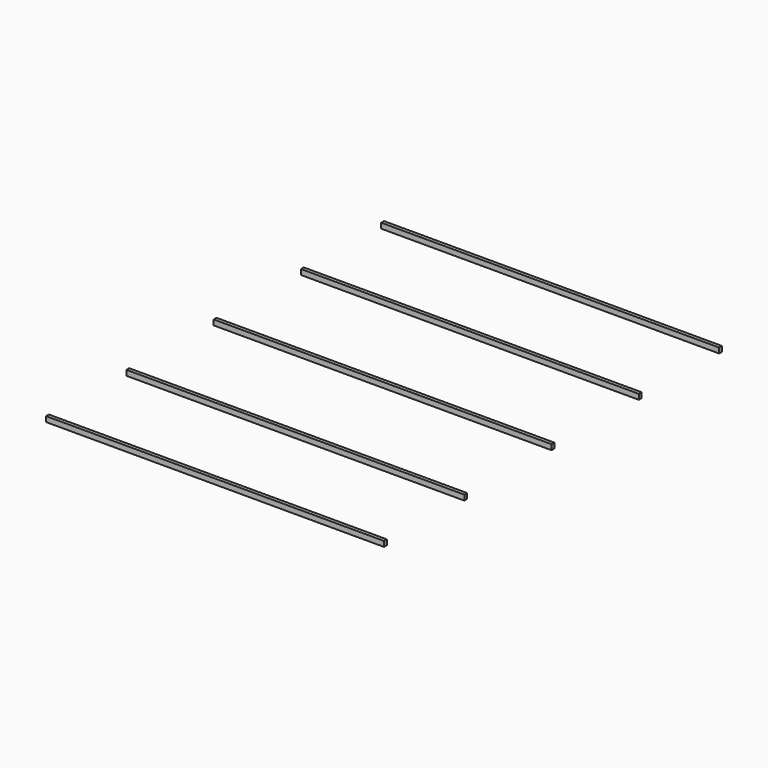
from build123d import *

# Parameters (mm, degrees)
F0_W     = 381
F0_H     = 4.2333333333
F0_W_2   = 25.4
F1_DEPTH = 6.35


with BuildPart() as f1:
    # F0 (on Top) → F1 (new body)
    with BuildSketch(Plane.XY):
        with Locations((0, 251.8833333333)):
            Rectangle(F0_W, F0_H)
        with Locations((203.2, 251.8833333333)):
            Rectangle(F0_W_2, F0_H)
    extrude(amount=F1_DEPTH)


with BuildPart() as f1b:
    # F0 (on Top) → F1, piece 2 (new body)
    with BuildSketch(Plane.XY):
        with Locations((203.2, 131.2333333333)):
            Rectangle(F0_W_2, F0_H)
        with Locations((0, 131.2333333333)):
            Rectangle(F0_W, F0_H)
    extrude(amount=F1_DEPTH)


with BuildPart() as f1c:
    # F0 (on Top) → F1, piece 3 (new body)
    with BuildSketch(Plane.XY):
        with Locations((203.2, 0)):
            Rectangle(F0_W_2, F0_H)
        Rectangle(F0_W, F0_H)
    extrude(amount=F1_DEPTH)


with BuildPart() as f1d:
    # F0 (on Top) → F1, piece 4 (new body)
    with BuildSketch(Plane.XY):
        with Locations((203.2, -131.2333333333)):
            Rectangle(F0_W_2, F0_H)
        with Locations((0, -131.2333333333)):
            Rectangle(F0_W, F0_H)
    extrude(amount=F1_DEPTH)


with BuildPart() as f1e:
    # F0 (on Top) → F1, piece 5 (new body)
    with BuildSketch(Plane.XY):
        with Locations((203.2, -251.8833333333)):
            Rectangle(F0_W_2, F0_H)
        with Locations((0, -251.8833333333)):
            Rectangle(F0_W, F0_H)
    extrude(amount=F1_DEPTH)


solid = Compound([f1.part, f1b.part, f1c.part, f1d.part, f1e.part])
